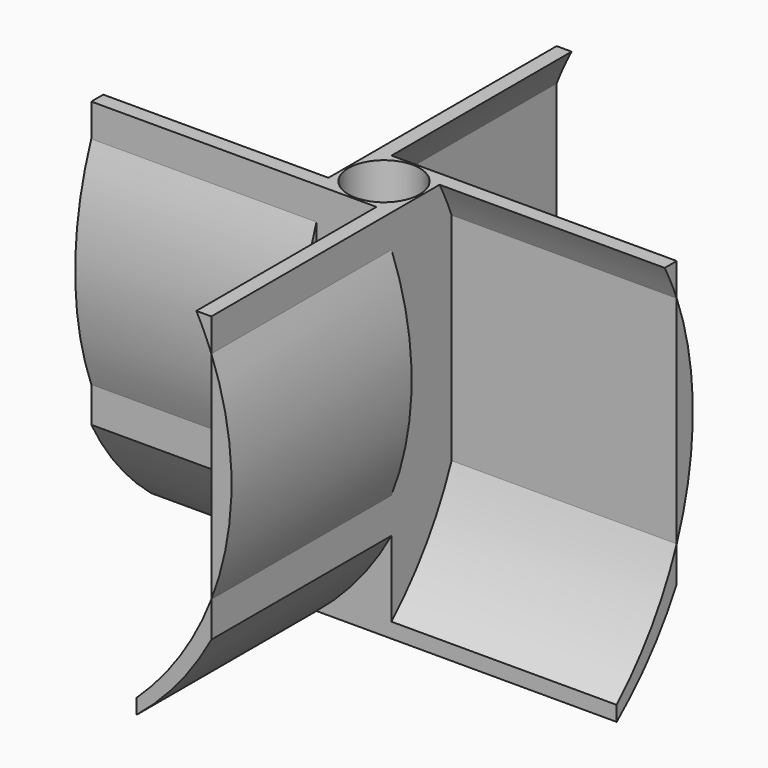
from build123d import *

# Parameters (mm, degrees)
F0_W     = 25.4
F0_H     = 25.4
F0_R     = 12.065
F1_DEPTH = 127
F6_DEPTH = 76.2
F7_DEPTH = 76.2
F8_DEPTH = 76.2
F9_DEPTH = 76.2


with BuildPart() as f1:
    # F0 (on Top) → F1 (new body)
    with BuildSketch(Plane.XY):
        Rectangle(F0_W, F0_H)
        Circle(F0_R, mode=Mode.SUBTRACT)
    extrude(amount=F1_DEPTH)

    # F2 (on face) → F6, piece 2 (join)
    with BuildSketch(Plane.YZ.offset(12.7)):
        with BuildLine():
            Line((-12.7, 5.08), (-12.7, 0))
            ThreePointArc((-12.7, 0), (1.5203011847, 14.096003508), (12.7, 30.7071026612))
            Line((12.7, 30.7071026612), (12.7, 42.7145954924))
            ThreePointArc((12.7, 42.7145954924), (2.1292313467, 22.460256229), (-12.7, 5.08))
        make_face()
        with BuildLine():
            Line((12.7, 115.8804951624), (12.7, 127))
            Line((12.7, 127), (7.62, 127))
            ThreePointArc((7.62, 127), (10.3273951692, 121.5167228804), (12.7, 115.8804951624))
        make_face()
    extrude(amount=F6_DEPTH)

    # F3 (on face) → F7 (join)
    with BuildSketch(Plane.XZ.offset(12.7)):
        with BuildLine():
            Line((-12.7, 5.08), (-12.7, 0))
            ThreePointArc((-12.7, 0), (1.5203011847, 14.096003508), (12.7, 30.7071026612))
            Line((12.7, 30.7071026612), (12.7, 42.7145954924))
            ThreePointArc((12.7, 42.7145954924), (2.1292313467, 22.460256229), (-12.7, 5.08))
        make_face()
        with BuildLine():
            Line((12.7, 115.8804951624), (12.7, 127))
            Line((12.7, 127), (7.62, 127))
            ThreePointArc((7.62, 127), (10.3273951692, 121.5167228804), (12.7, 115.8804951624))
        make_face()
    extrude(amount=F7_DEPTH)

    # F4 (on face) → F8, piece 2 (join)
    with BuildSketch(Plane(origin=(-12.7, 0, 0), x_dir=(0, -1, 0), z_dir=(-1, 0, 0))):
        with BuildLine():
            ThreePointArc((12.7, 42.7145954924), (2.1292313467, 22.460256229), (-12.7, 5.08))
            Line((-12.7, 5.08), (-12.7, 0))
            ThreePointArc((-12.7, 0), (1.5203011847, 14.096003508), (12.7, 30.7071026612))
            Line((12.7, 30.7071026612), (12.7, 42.7145954924))
        make_face()
        with BuildLine():
            ThreePointArc((7.62, 127), (10.3273951692, 121.5167228804), (12.7, 115.8804951624))
            Line((12.7, 115.8804951624), (12.7, 127))
            Line((12.7, 127), (7.62, 127))
        make_face()
    extrude(amount=F8_DEPTH)

    # F5 (on face) → F9, piece 2 (join)
    with BuildSketch(Plane(origin=(0, 12.7, 0), x_dir=(-1, 0, 0), z_dir=(0, 1, 0))):
        with BuildLine():
            Line((-12.7, 5.08), (-12.7, 0))
            ThreePointArc((-12.7, 0), (1.5203011847, 14.096003508), (12.7, 30.7071026612))
            Line((12.7, 30.7071026612), (12.7, 42.7145954924))
            ThreePointArc((12.7, 42.7145954924), (2.1292313467, 22.460256229), (-12.7, 5.08))
        make_face()
        with BuildLine():
            Line((12.7, 115.8804951624), (12.7, 127))
            Line((12.7, 127), (7.62, 127))
            ThreePointArc((7.62, 127), (10.3273951692, 121.5167228804), (12.7, 115.8804951624))
        make_face()
    extrude(amount=F9_DEPTH)


with BuildPart() as f6:
    # F2 (on face) → F6 (new body)
    with BuildSketch(Plane.YZ.offset(12.7)):
        with BuildLine():
            Line((12.7, 115.8804951624), (12.7, 42.7145954924))
            ThreePointArc((12.7, 42.7145954924), (19.5147280356, 79.2975453274), (12.7, 115.8804951624))
        make_face()
    extrude(amount=F6_DEPTH)


with BuildPart() as f7:
    # F3 (on face) → F7, piece 2 (new body)
    with BuildSketch(Plane.XZ.offset(12.7)):
        with BuildLine():
            Line((12.7, 115.8804951624), (12.7, 42.7145954924))
            ThreePointArc((12.7, 42.7145954924), (19.5147280356, 79.2975453274), (12.7, 115.8804951624))
        make_face()
    extrude(amount=F7_DEPTH)


with BuildPart() as f8:
    # F4 (on face) → F8 (new body)
    with BuildSketch(Plane(origin=(-12.7, 0, 0), x_dir=(0, -1, 0), z_dir=(-1, 0, 0))):
        with BuildLine():
            Line((12.7, 115.8804951624), (12.7, 42.7145954924))
            ThreePointArc((12.7, 42.7145954924), (19.5147280356, 79.2975453274), (12.7, 115.8804951624))
        make_face()
    extrude(amount=F8_DEPTH)


with BuildPart() as f9:
    # F5 (on face) → F9 (new body)
    with BuildSketch(Plane(origin=(0, 12.7, 0), x_dir=(-1, 0, 0), z_dir=(0, 1, 0))):
        with BuildLine():
            Line((12.7, 115.8804951624), (12.7, 42.7145954924))
            ThreePointArc((12.7, 42.7145954924), (19.5147280356, 79.2975453274), (12.7, 115.8804951624))
        make_face()
    extrude(amount=F9_DEPTH)


solid = Compound([f1.part, f6.part, f7.part, f8.part, f9.part])
